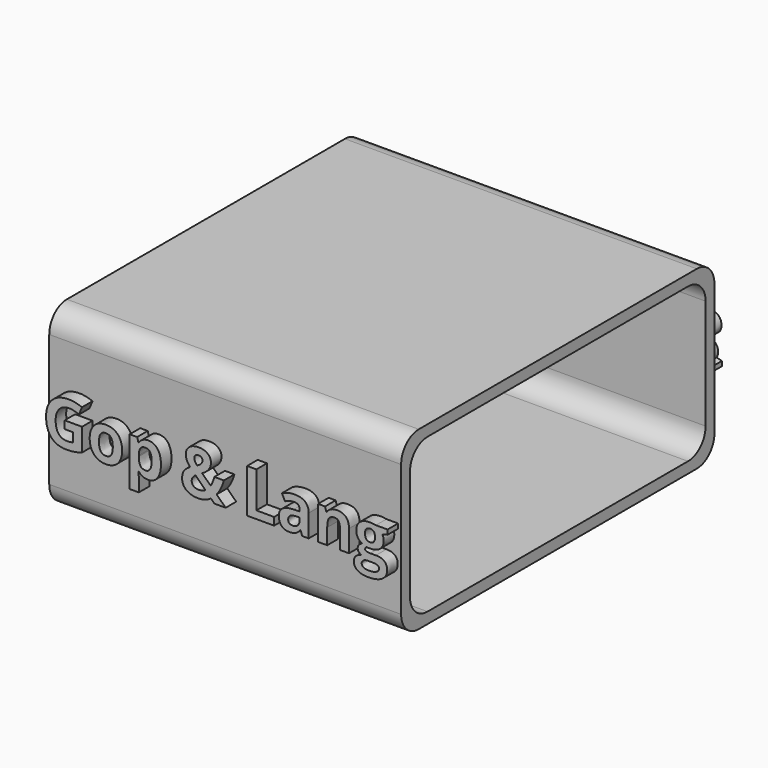
from build123d import *

# Parameters (mm, degrees)
F0_W         = 80
F0_H         = 89.0232706736
F1_DEPTH     = 40
F2_T         = -2.5
F3_R         = 5
F4_R         = 5
F5_R         = 5
F6_TEXT_SIZE = 13.9443113262
F7_DEPTH     = 3
F8_R         = 5
F9_R         = 5
F10_R        = 5
F12_COUNT    = 2


# Not quite as in the source:
# - Text() gives the source's letters only with a copy of the font that has no kerning and outlines rounded to 1/6400 em; it was checked with that copy


with BuildPart() as f1:
    # F0 (on Top) → F1 (new body)
    with BuildSketch(Plane.XY):
        Rectangle(F0_W, F0_H)
    extrude(amount=F1_DEPTH)

    # F2
    f2_openings = [f1.faces().sort_by_distance(p)[0] for p in [
        (40, 0, 20),
    ]]
    offset(amount=F2_T, openings=f2_openings)

    # F3
    f3_edges = [f1.edges().sort_by_distance(p)[0] for p in [
        (0, -44.511635, 40),
    ]]
    fillet(f3_edges, radius=F3_R)

    # F4
    f4_edges = [f1.edges().sort_by_distance(p)[0] for p in [
        (0, -44.511635, 0),
    ]]
    fillet(f4_edges, radius=F4_R)

    # F5
    f5_edges = [f1.edges().sort_by_distance(p)[0] for p in [
        (0, 44.511635, 0),
        (0, 44.511635, 40),
    ]]
    fillet(f5_edges, radius=F5_R)

    # F6 (on face) → F7 (join)
    with BuildSketch(Plane.XZ.offset(44.5116353368)):
        with Locations((-39.1336204484, 15.3600936756)):
            Text('Gop & Lang', F6_TEXT_SIZE, font='Open Sans', font_style=FontStyle.BOLD, text_align=(TextAlign.LEFT, TextAlign.BOTTOM))
    extrude(amount=F7_DEPTH)

    # F8
    f8_edges = [f1.edges().sort_by_distance(p)[0] for p in [
        (1.25, -42.011635, 37.5),
        (1.25, -42.011635, 2.5),
    ]]
    fillet(f8_edges, radius=F8_R)

    # F9
    f9_edges = [f1.edges().sort_by_distance(p)[0] for p in [
        (1.25, 42.011635, 37.5),
    ]]
    fillet(f9_edges, radius=F9_R)

    # F10
    f10_edges = [f1.edges().sort_by_distance(p)[0] for p in [
        (1.25, 42.011635, 2.5),
    ]]
    fillet(f10_edges, radius=F10_R)


with BuildPart() as f12_1:
    # F12: instance of F1
    add(f1.part.rotate(Axis((-40, 0, 20), (1, 0, 0)), 1 * 360 / F12_COUNT))


solid = Compound([f1.part, f12_1.part])
